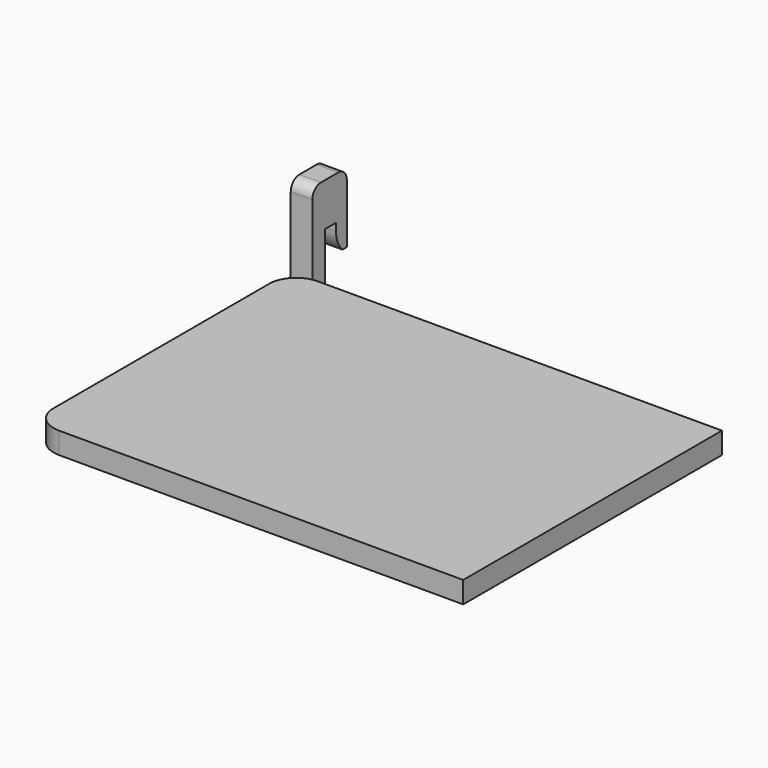
from build123d import *

# Parameters (mm, degrees)
F2_W        = 4
F2_H        = 11
F3_DEPTH    = 4
F4_W        = 4
F4_H        = 3
F5_DEPTH    = 25
F6_W        = 4
F6_H        = 2.5
F7_DEPTH    = 5
F8_SIZE2    = 1
F8_SIZE     = 1.5
F9_T1_DEPTH = 16.8535710714
F10_R       = 5
F11_W       = 4
F11_H       = 4
F11_W_2     = 76
F12_DEPTH   = 60
F14_W       = 12.6825077459
F14_H       = 13.7545838952
F15_DEPTH   = 25
F16_R       = 2
F17_R       = 5
F19_W       = 20.4623111058
F19_H       = 23.2868297026
F20_DEPTH   = 25
F21_R       = 1.99999


# Not quite as in the source:
# - a fillet or chamfer that OpenCascade refuses, or shapes differently, is made with other operations: its cross-section is extruded or revolved along the edge and cut away or added
# - a fillet or chamfer is up to 0.001 mm smaller than in the source, because OpenCascade refuses the exact size


with BuildPart() as f3:
    # F2 (on Front) → F3 (new body, symmetric)
    with BuildSketch(Plane.XZ):
        with Locations((-16.0614851415, 19.6203391254)):
            Rectangle(F2_W, F2_H)
    extrude(amount=F3_DEPTH, both=True)

    # F4 (on face) → F5 (join)
    with BuildSketch(Plane(origin=(0, 0, 14.1203391254), x_dir=(1, 0, 0), z_dir=(0, 0, -1))):
        with Locations((-16.0614851415, 2.5)):
            Rectangle(F4_W, F4_H)
    extrude(amount=F5_DEPTH)

    # F6 (on face) → F7 (join)
    with BuildSketch(Plane(origin=(0, 0, 14.1203391254), x_dir=(1, 0, 0), z_dir=(0, 0, -1))):
        with Locations((-16.0614851415, -2.75)):
            Rectangle(F6_W, F6_H)
    extrude(amount=F7_DEPTH)

    # F8
    f8_edges = [f3.edges().sort_by_distance(p)[0] for p in [
        (-16.061485, 1.5, 9.120339),
    ]]
    f8_side = f3.faces().sort_by_distance((-16.061485, 2.75, 9.120339))[0]
    chamfer(f8_edges, length=F8_SIZE, length2=F8_SIZE2, reference=f8_side)

    # F9: fillet of radius 5 on 1 edges, made by hand

    # F9_s2 → F9_t1 (cut)
    with BuildSketch(Plane.YZ.offset(-24.4882706772)):
        with BuildLine():
            ThreePointArc((1.5, 12.6910533397), (1.8902277714, 10.7545616666), (3, 9.1203391254))
            Line((3, 9.1203391254), (1.5, 10.1203391254))
            Line((1.5, 10.1203391254), (1.5, 12.6910533397))
        make_face()
    extrude(amount=F9_T1_DEPTH, mode=Mode.SUBTRACT)

    # F10
    f10_edges = [f3.edges().sort_by_distance(p)[0] for p in [
        (-16.061485, 4, 25.120339),
    ]]
    fillet(f10_edges, radius=F10_R)

    # F14 (on offset) → F15 (cut)
    with BuildSketch(Plane(origin=(0, 0, -2.3372200429), x_dir=(1, 0, 0), z_dir=(0, 0, -1))):
        with Locations((-17.142616678, -0.0888193026)):
            Rectangle(F14_W, F14_H)
    extrude(amount=F15_DEPTH, mode=Mode.SUBTRACT)

    # F16
    f16_edges = [f3.edges().sort_by_distance(p)[0] for p in [
        (-16.061485, -4, 25.120339),
    ]]
    fillet(f16_edges, radius=F16_R)

    # F19 (on offset) → F20 (cut)
    with BuildSketch(Plane.XY.offset(22.1203391254)):
        with Locations((-13.2027346408, 1.5548248775)):
            Rectangle(F19_W, F19_H)
    extrude(amount=F20_DEPTH, mode=Mode.SUBTRACT)

    # F21 (radius 2 in the source; OpenCascade refuses exactly that, so slightly less here)
    f21_edges = [f3.edges().sort_by_distance(p)[0] for p in [
        (-16.061485, -4, 22.120339),
        (-16.061485, 3.582576, 22.120339),
    ]]
    fillet(f21_edges, radius=F21_R)


with BuildPart() as f12:
    # F11 (on face) → F12 (new body)
    with BuildSketch(Plane.XZ.offset(4)):
        with Locations((-16.0614851415, 5.1203391254)):
            Rectangle(F11_W, F11_H)
        with Locations((23.9385148585, 5.1203391254)):
            Rectangle(F11_W_2, F11_H)
    extrude(amount=F12_DEPTH)

    # F17
    f17_edges = [f12.edges().sort_by_distance(p)[0] for p in [
        (-18.061485, -4, 5.120339),
        (-18.061485, -64, 5.120339),
    ]]
    fillet(f17_edges, radius=F17_R)


solid = Compound([f3.part, f12.part])
